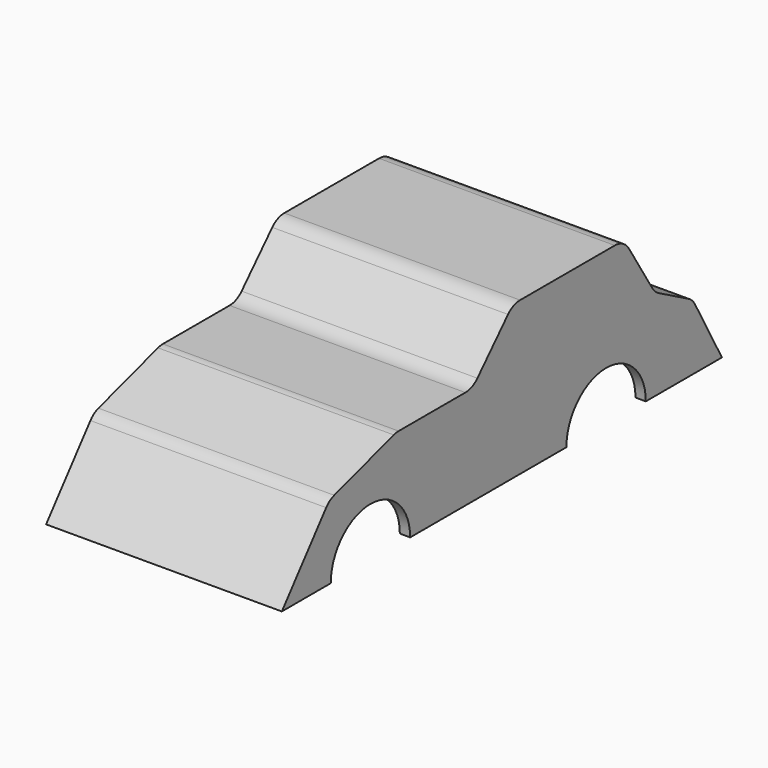
from build123d import *

# Parameters (mm, degrees)
F1_DEPTH = 57
F2_T     = -2.5
F3_R     = 5
F4_R     = 5


with BuildPart() as f1:
    # F0 (on Right) → F1 (new body)
    with BuildSketch(Plane.YZ):
        with BuildLine():
            ThreePointArc((23.7267759775, 0), (35.7267759775, 12), (47.7267759775, 0))
            Line((47.7267759775, 0), (70.7267759775, 0))
            Line((70.7267759775, 0), (61.8750043213, 15.9051734954))
            Line((61.8750043213, 15.9051734954), (50.431035459, 22.1120696515))
            Line((50.431035459, 22.1120696515), (41.1206930876, 37))
            Line((41.1206930876, 37), (7.5646545738, 37))
            Line((7.5646545738, 37), (-4.6551725827, 24.0517258644))
            Line((-4.6551725827, 24.0517258644), (-27.737069875, 24.0517258644))
            Line((-27.737069875, 24.0517258644), (-47.9094833136, 17.8448278457))
            Line((-47.9094833136, 17.8448278457), (-62.2732240225, 0))
            Line((-62.2732240225, 0), (-47.4932240225, 0))
            ThreePointArc((-47.4932240225, 0), (-35.4932240225, 12), (-23.4932240225, 0))
            Line((-23.4932240225, 0), (23.7267759775, 0))
        make_face()
    extrude(amount=F1_DEPTH)

    # F2
    f2_openings = [f1.faces().sort_by_distance(p)[0] for p in [
        (28.5, 0.116776, 0),
        (28.5, -35.493224, 12),
        (28.5, 35.726776, 12),
        (28.5, 59.226776, 0),
        (28.5, -54.883224, 0),
    ]]
    offset(amount=F2_T, openings=f2_openings, kind=Kind.INTERSECTION)

    # F3
    f3_edges = [f1.edges().sort_by_distance(p)[0] for p in [
        (28.5, -47.909483, 17.844828),
        (28.5, -27.73707, 24.051726),
        (28.5, -4.655173, 24.051726),
        (28.5, 7.564655, 37),
        (28.5, 41.120693, 37),
        (28.5, 50.431035, 22.11207),
        (28.5, 61.875004, 15.905173),
    ]]
    fillet(f3_edges, radius=F3_R)

    # F4
    f4_edges = [f1.edges().sort_by_distance(p)[0] for p in [
        (28.5, -46.44224, 15.68062),
        (28.5, -27.361151, 21.551726),
        (28.5, -3.577006, 21.551726),
        (28.5, 8.642822, 34.5),
        (28.5, 39.735499, 34.5),
        (28.5, 48.660441, 20.228354),
        (28.5, 60.044051, 14.054195),
    ]]
    fillet(f4_edges, radius=F4_R)


solid = f1.part
